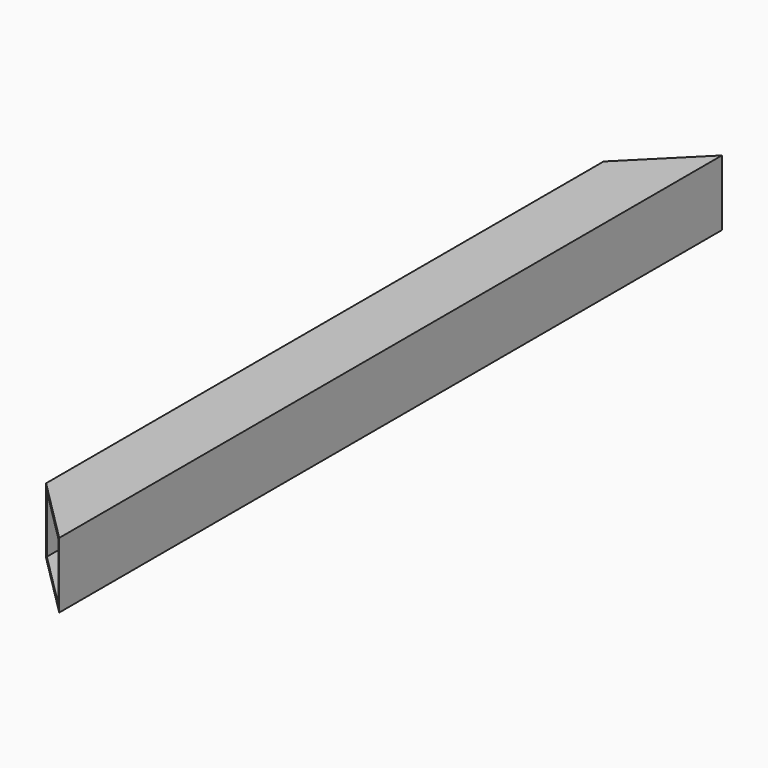
from build123d import *

# Parameters (mm, degrees)
F0_W        = 50
F0_H        = 50
F0_W_2      = 44
F0_H_2      = 44
F1_DEPTH    = 630
F2_T1_DEPTH = 307.1682987966
F3_T1_DEPTH = 307.1682987966


# Not quite as in the source:
# - a fillet or chamfer that OpenCascade refuses, or shapes differently, is made with other operations: its cross-section is extruded or revolved along the edge and cut away or added


with BuildPart() as f1:
    # F0 (on Front) → F1 (new body)
    with BuildSketch(Plane.XZ):
        Rectangle(F0_W, F0_H)
        Rectangle(F0_W_2, F0_H_2, mode=Mode.SUBTRACT)
    extrude(amount=F1_DEPTH)

    # F2: chamfer of 50 on 1 edges, made by hand

    # F2_s2 → F2_t1 (cut)
    with BuildSketch(Plane.XY.offset(-153.5841493983)):
        Polygon((-25, -580), (25, -630), (-25, -630), align=None)
    extrude(amount=F2_T1_DEPTH, mode=Mode.SUBTRACT)

    # F3: chamfer of 50 on 1 edges, made by hand

    # F3_s2 → F3_t1 (cut)
    with BuildSketch(Plane.XY.offset(-153.5841493983)):
        Polygon((25, 0), (-25, -50), (-25, 0), align=None)
    extrude(amount=F3_T1_DEPTH, mode=Mode.SUBTRACT)


solid = f1.part
